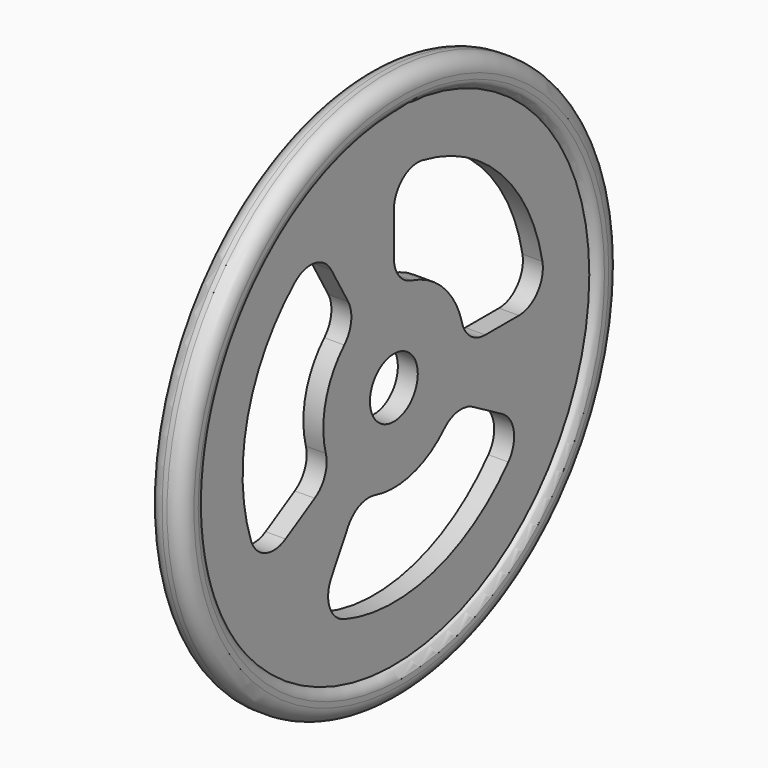
from build123d import *

# Parameters (mm, degrees)
F0_R     = 24.5
F0_R_2   = 3
F1_DEPTH = 1
F0_R_3   = 27.5
F2_DEPTH = 1.75
F3_R     = 1.5
F5_R     = 3


# Not quite as in the source:
# - a fillet or chamfer that OpenCascade refuses, or shapes differently, is made with other operations: its cross-section is extruded or revolved along the edge and cut away or added


with BuildPart() as f1:
    # F0 (on Right) → F1 (new body, symmetric)
    with BuildSketch(Plane.YZ):
        Circle(F0_R)
        with BuildLine():
            ThreePointArc((0, 18.9637232794), (13.4093773274, 13.4093773274), (18.9637232794, 0))
            ThreePointArc((18.9637232794, 0), (18.3175500781, -4.9081727508), (16.4230661103, -9.4818616397))
            ThreePointArc((16.4230661103, -9.4818616397), (4.9081727508, -18.3175500781), (-9.4818616397, -16.4230661103))
            ThreePointArc((-9.4818616397, -16.4230661103), (-13.4093773274, -13.4093773274), (-16.4230661103, -9.4818616397))
            ThreePointArc((-16.4230661103, -9.4818616397), (-18.3175500781, 4.9081727508), (-9.4818616397, 16.4230661103))
            ThreePointArc((-9.4818616397, 16.4230661103), (-4.9081727508, 18.3175500781), (0, 18.9637232794))
        make_face(mode=Mode.SUBTRACT)
        with BuildLine():
            ThreePointArc((7.6604867484, -4.4227840863), (8.5441627462, -2.2894015078), (8.8455681727, 0))
            ThreePointArc((8.8455681727, 0), (6.2547612383, 6.2547612383), (0, 8.8455681727))
            ThreePointArc((0, 8.8455681727), (-2.2894015078, 8.5441627462), (-4.4227840863, 7.6604867484))
            ThreePointArc((-4.4227840863, 7.6604867484), (-8.5441627462, 2.2894015078), (-7.6604867484, -4.4227840863))
            ThreePointArc((-7.6604867484, -4.4227840863), (-6.2547612383, -6.2547612383), (-4.4227840863, -7.6604867484))
            ThreePointArc((-4.4227840863, -7.6604867484), (2.2894015078, -8.5441627462), (7.6604867484, -4.4227840863))
        make_face()
        Circle(F0_R_2, mode=Mode.SUBTRACT)
        with BuildLine():
            Line((0, 8.8455681727), (0, 18.9637232794))
            ThreePointArc((0, 18.9637232794), (-4.9081727508, 18.3175500781), (-9.4818616397, 16.4230661103))
            Line((-9.4818616397, 16.4230661103), (-4.4227840863, 7.6604867484))
            ThreePointArc((-4.4227840863, 7.6604867484), (-2.2894015078, 8.5441627462), (0, 8.8455681727))
        make_face()
        with BuildLine():
            ThreePointArc((-16.4230661103, -9.4818616397), (-13.4093773274, -13.4093773274), (-9.4818616397, -16.4230661103))
            Line((-9.4818616397, -16.4230661103), (-4.4227840863, -7.6604867484))
            ThreePointArc((-4.4227840863, -7.6604867484), (-6.2547612383, -6.2547612383), (-7.6604867484, -4.4227840863))
            Line((-7.6604867484, -4.4227840863), (-16.4230661103, -9.4818616397))
        make_face()
        with BuildLine():
            ThreePointArc((16.4230661103, -9.4818616397), (18.3175500781, -4.9081727508), (18.9637232794, 0))
            Line((18.9637232794, 0), (8.8455681727, 0))
            ThreePointArc((8.8455681727, 0), (8.5441627462, -2.2894015078), (7.6604867484, -4.4227840863))
            Line((7.6604867484, -4.4227840863), (16.4230661103, -9.4818616397))
        make_face()
    extrude(amount=F1_DEPTH, both=True)

    # F0 (on Right) → F2 (join, symmetric)
    with BuildSketch(Plane.YZ):
        Circle(F0_R_3)
        Circle(F0_R, mode=Mode.SUBTRACT)
    extrude(amount=F2_DEPTH, both=True)

    # F3
    f3_edges = [f1.edges().sort_by_distance(p)[0] for p in [
        (-1.75, -27.5, 0),
        (1.75, -27.5, 0),
    ]]
    fillet(f3_edges, radius=F3_R)

    # F4: fillet of radius 1 on 2 edges, made by hand

    # F4_s1 → F4_t2 (revolve, cut)
    with BuildSketch(Plane.XY):
        with BuildLine():
            ThreePointArc((1.75, 25.4682458366), (1.540569415, 24.8558734009), (1, 24.5))
            Line((1, 24.5), (1.75, 24.5))
            Line((1.75, 24.5), (1.75, 25.4682458366))
        make_face()
    revolve(axis=Axis((1.75, 0, 0), (1, 0, 0)), mode=Mode.SUBTRACT)

    # F4_s3 → F4_t4 (revolve, cut)
    with BuildSketch(Plane.XY):
        with BuildLine():
            ThreePointArc((-1.75, 25.4682458366), (-1.540569415, 24.8558734009), (-1, 24.5))
            Line((-1, 24.5), (-1.75, 24.5))
            Line((-1.75, 24.5), (-1.75, 25.4682458366))
        make_face()
    revolve(axis=Axis((-1.75, 0, 0), (1, 0, 0)), mode=Mode.SUBTRACT)

    # F5
    f5_edges = [f1.edges().sort_by_distance(p)[0] for p in [
        (0, -16.423066, -9.481862),
        (0, -7.660487, -4.422784),
        (0, -4.422784, 7.660487),
        (0, 0, 18.963723),
        (0, -9.481862, 16.423066),
        (0, -4.422784, -7.660487),
        (0, 7.660487, -4.422784),
        (0, 0, 8.845568),
        (0, 8.845568, 0),
        (0, -9.481862, -16.423066),
        (0, 16.423066, -9.481862),
        (0, 18.963723, 0),
    ]]
    fillet(f5_edges, radius=F5_R)


solid = f1.part
